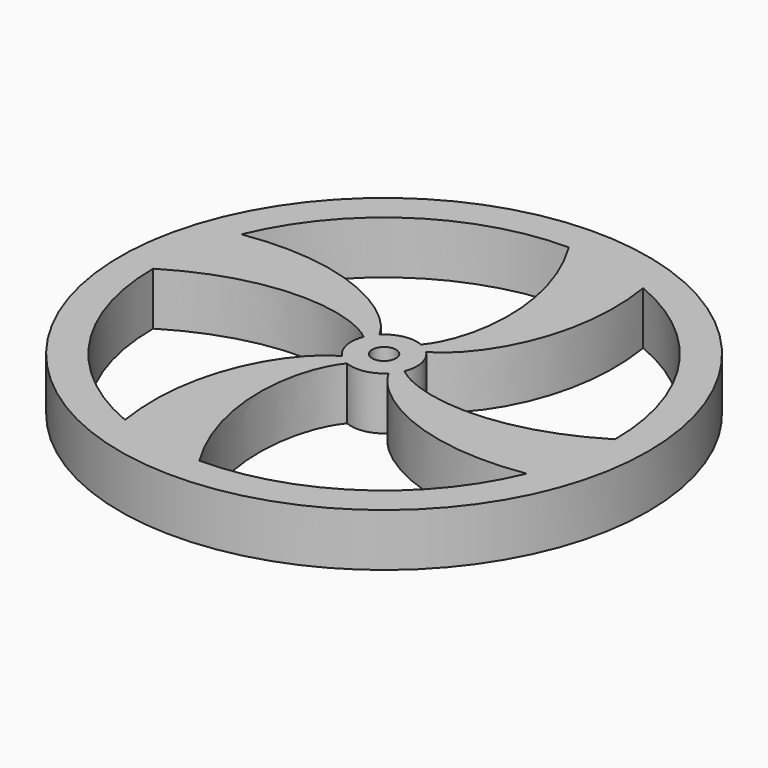
from build123d import *

# Parameters (mm, degrees)
F0_R     = 20
F0_R_2   = 0.9
F1_DEPTH = 4


with BuildPart() as f1:
    # F0 (on Top) → F1 (new body)
    with BuildSketch(Plane.XY):
        Circle(F0_R)
        with BuildLine():
            ThreePointArc((-16.1673680712, 6.6982243655), (-9.7219101416, 14.5510983502), (0, 17.5))
            add(Edge.make_bspline(
                [(0, 17.5), (4.0351947292, 10.8956713768), (2.8402573141, 4.5637440123), (0.9567085809, 2.3096988313)],
                knots=[0, 0, 0, 0, 0.6747802814, 0.6747802814, 0.6747802814, 0.6747802814], degree=3))
            add(Edge.make_bspline(
                [(1.05334234, 1.483872858), (1.0137768965, 1.7486550509), (0.9849575618, 2.0237015142), (0.9567085809, 2.3096988313)],
                knots=[0.9279449305, 0.9279449305, 0.9279449305, 0.9279449305, 1, 1, 1, 1], degree=3))
            add(Edge.make_bspline(
                [(1.7677669525, 1.7677669535), (1.7677118309, 1.7677381162), (1.5223929609, 1.6394048238), (1.2852910821, 1.5468737836), (1.0533423393, 1.4838728598)],
                knots=[0.6747713742, 0.6747713742, 0.6747713742, 0.6747713742, 0.6747856641, 0.7383691109, 0.7383691109, 0.7383691109, 0.7383691109], degree=3))
            add(Edge.make_bspline(
                [(1.76803561, 1.7679075162), (1.7679460564, 1.7678606572), (1.7678565039, 1.7678138029), (1.7677669525, 1.7677669535)],
                knots=[0.6747481586, 0.6747481586, 0.6747481586, 0.6747481586, 0.6747713742, 0.6747713742, 0.6747713742, 0.6747713742], degree=3))
            add(Edge.make_bspline(
                [(6.6984395879, 16.1672789018), (7.8983091219, 8.521720501), (4.3708601286, 3.1298383292), (1.76803561, 1.7679075162)],
                knots=[0, 0, 0, 0, 0.6747481586, 0.6747481586, 0.6747481586, 0.6747481586], degree=3))
            ThreePointArc((6.6984395879, 16.1672789018), (14.5511630598, 9.721813288), (17.5, 0))
            add(Edge.make_bspline(
                [(17.5, 0), (10.8956713768, -4.0351947292), (4.5637440123, -2.8402573141), (2.3096988313, -0.9567085809)],
                knots=[0, 0, 0, 0, 0.6747802814, 0.6747802814, 0.6747802814, 0.6747802814], degree=3))
            add(Edge.make_bspline(
                [(1.4839305002, -1.0533337269), (1.7486949687, -1.0137727139), (2.0237222677, -0.9849555119), (2.3096988313, -0.9567085809)],
                knots=[0.9279501592, 0.9279501592, 0.9279501592, 0.9279501592, 1, 1, 1, 1], degree=3))
            add(Edge.make_bspline(
                [(1.767766953, -1.767766953), (1.7677424454, -1.767720101), (1.639424724, -1.5224005371), (1.5469125425, -1.2852951635), (1.483930502, -1.0533337262)],
                knots=[0.6747683451, 0.6747683451, 0.6747683451, 0.6747683451, 0.674780491, 0.7383651842, 0.7383651842, 0.7383651842, 0.7383651842], degree=3))
            add(Edge.make_bspline(
                [(1.7679075011, -1.7680356179), (1.767860647, -1.7679460618), (1.7678137976, -1.7678565068), (1.767766953, -1.767766953)],
                knots=[0.6747451292, 0.6747451292, 0.6747451292, 0.6747451292, 0.6747683451, 0.6747683451, 0.6747683451, 0.6747683451], degree=3))
            add(Edge.make_bspline(
                [(16.1673680713, -6.6982243654), (8.5218439975, -7.8980885198), (3.1296734519, -4.3708895859), (1.7679075011, -1.7680356179)],
                knots=[0, 0, 0, 0, 0.6747451292, 0.6747451292, 0.6747451292, 0.6747451292], degree=3))
            ThreePointArc((16.1673680713, -6.6982243654), (9.7219101417, -14.5510983502), (0, -17.5))
            add(Edge.make_bspline(
                [(0, -17.5), (-4.0351947292, -10.8956713768), (-2.8402573141, -4.5637440123), (-0.9567085809, -2.3096988313)],
                knots=[0, 0, 0, 0, 0.6747802814, 0.6747802814, 0.6747802814, 0.6747802814], degree=3))
            add(Edge.make_bspline(
                [(-1.0533337269, -1.4839305003), (-1.0137727139, -1.7486949687), (-0.9849555119, -2.0237222677), (-0.9567085809, -2.3096988313)],
                knots=[0.9279501592, 0.9279501592, 0.9279501592, 0.9279501592, 1, 1, 1, 1], degree=3))
            add(Edge.make_bspline(
                [(-1.767766953, -1.767766953), (-1.7677201011, -1.7677424454), (-1.5224005372, -1.639424724), (-1.2852951635, -1.5469125425), (-1.0533337262, -1.483930502)],
                knots=[0.6747683451, 0.6747683451, 0.6747683451, 0.6747683451, 0.674780491, 0.7383651842, 0.7383651842, 0.7383651842, 0.7383651842], degree=3))
            add(Edge.make_bspline(
                [(-1.7680356179, -1.7679075011), (-1.7679460618, -1.767860647), (-1.7678565068, -1.7678137976), (-1.767766953, -1.767766953)],
                knots=[0.6747451293, 0.6747451293, 0.6747451293, 0.6747451293, 0.6747683451, 0.6747683451, 0.6747683451, 0.6747683451], degree=3))
            add(Edge.make_bspline(
                [(-6.6982243654, -16.1673680712), (-7.8980885199, -8.5218439973), (-4.3708895859, -3.1296734518), (-1.7680356179, -1.7679075011)],
                knots=[0, 0, 0, 0, 0.6747451293, 0.6747451293, 0.6747451293, 0.6747451293], degree=3))
            ThreePointArc((-6.6982243654, -16.1673680712), (-14.5510983502, -9.7219101417), (-17.5, 0))
            add(Edge.make_bspline(
                [(-17.5, 0), (-10.8956713768, 4.0351947292), (-4.5637440123, 2.8402573141), (-2.3096988313, 0.9567085809)],
                knots=[0, 0, 0, 0, 0.6747802814, 0.6747802814, 0.6747802814, 0.6747802814], degree=3))
            add(Edge.make_bspline(
                [(-1.4839305003, 1.0533337269), (-1.7486949687, 1.0137727139), (-2.0237222677, 0.9849555119), (-2.3096988313, 0.9567085809)],
                knots=[0.9279501592, 0.9279501592, 0.9279501592, 0.9279501592, 1, 1, 1, 1], degree=3))
            add(Edge.make_bspline(
                [(-1.767766953, 1.767766953), (-1.7677424454, 1.7677201011), (-1.6394247241, 1.5224005372), (-1.5469125425, 1.2852951636), (-1.4839305021, 1.0533337262)],
                knots=[0.6747683451, 0.6747683451, 0.6747683451, 0.6747683451, 0.674780491, 0.7383651842, 0.7383651842, 0.7383651842, 0.7383651842], degree=3))
            add(Edge.make_bspline(
                [(-16.1673680712, 6.6982243655), (-8.5215809386, 7.8981298036), (-3.1293023988, 4.3706468604), (-1.767766953, 1.767766953)],
                knots=[0, 0, 0, 0, 0.6747683451, 0.6747683451, 0.6747683451, 0.6747683451], degree=3))
        make_face(mode=Mode.SUBTRACT)
        with BuildLine():
            add(Edge.make_bspline(
                [(1.05334234, 1.483872858), (1.0137768965, 1.7486550509), (0.9849575618, 2.0237015142), (0.9567085809, 2.3096988313)],
                knots=[0.9279449305, 0.9279449305, 0.9279449305, 0.9279449305, 1, 1, 1, 1], degree=3))
            add(Edge.make_bspline(
                [(0.9567085809, 2.3096988313), (0.5925556194, 1.873916516), (0.202663868, 1.5905565475), (-0.2170414882, 1.3992266891)],
                knots=[0.6747802814, 0.6747802814, 0.6747802814, 0.6747802814, 0.8052378764, 0.8052378764, 0.8052378764, 0.8052378764], degree=3))
            add(Edge.make_bspline(
                [(1.0533423393, 1.4838728598), (0.6188058723, 1.3658459262), (0.2021683226, 1.3513874939), (-0.2170414882, 1.3992266891)],
                knots=[0.7383691109, 0.7383691109, 0.7383691109, 0.7383691109, 0.8574873522, 0.8574873522, 0.8574873522, 0.8574873522], degree=3))
        make_face()
        with BuildLine():
            add(Edge.make_bspline(
                [(0.9567085809, 2.3096988313), (0.5925556194, 1.873916516), (0.202663868, 1.5905565475), (-0.2170414882, 1.3992266891)],
                knots=[0.6747802814, 0.6747802814, 0.6747802814, 0.6747802814, 0.8052378764, 0.8052378764, 0.8052378764, 0.8052378764], degree=3))
            ThreePointArc((0.9567085809, 2.3096988313), (-0.4877258051, 2.451963201), (-1.767766953, 1.767766953))
            add(Edge.make_bspline(
                [(-0.2170414882, 1.3992266891), (-0.7185826414, 1.4564613351), (-1.2238056379, 1.6028665997), (-1.767766953, 1.767766953)],
                knots=[0.8574873522, 0.8574873522, 0.8574873522, 0.8574873522, 1, 1, 1, 1], degree=3))
        make_face()
        with BuildLine():
            add(Edge.make_bspline(
                [(-0.2170414882, 1.3992266891), (-0.7185826414, 1.4564613351), (-1.2238056379, 1.6028665997), (-1.767766953, 1.767766953)],
                knots=[0.8574873522, 0.8574873522, 0.8574873522, 0.8574873522, 1, 1, 1, 1], degree=3))
            add(Edge.make_bspline(
                [(-1.767766953, 1.767766953), (-1.7677424454, 1.7677201011), (-1.6394247241, 1.5224005372), (-1.5469125425, 1.2852951636), (-1.4839305021, 1.0533337262)],
                knots=[0.6747683451, 0.6747683451, 0.6747683451, 0.6747683451, 0.674780491, 0.7383651842, 0.7383651842, 0.7383651842, 0.7383651842], degree=3))
            add(Edge.make_bspline(
                [(-0.2170414882, 1.3992266891), (-0.6118287934, 1.21925615), (-1.0329947036, 1.1207123938), (-1.4839305003, 1.0533337269)],
                knots=[0.8052378764, 0.8052378764, 0.8052378764, 0.8052378764, 0.9279501592, 0.9279501592, 0.9279501592, 0.9279501592], degree=3))
        make_face()
        with BuildLine():
            add(Edge.make_bspline(
                [(1.0533423393, 1.4838728598), (0.6188058723, 1.3658459262), (0.2021683226, 1.3513874939), (-0.2170414882, 1.3992266891)],
                knots=[0.7383691109, 0.7383691109, 0.7383691109, 0.7383691109, 0.8574873522, 0.8574873522, 0.8574873522, 0.8574873522], degree=3))
            add(Edge.make_bspline(
                [(-0.2170414882, 1.3992266891), (-0.6118287934, 1.21925615), (-1.0329947036, 1.1207123938), (-1.4839305003, 1.0533337269)],
                knots=[0.8052378764, 0.8052378764, 0.8052378764, 0.8052378764, 0.9279501592, 0.9279501592, 0.9279501592, 0.9279501592], degree=3))
            add(Edge.make_bspline(
                [(-1.4839305021, 1.0533337262), (-1.3659750292, 0.6189063747), (-1.3515357612, 0.2023627588), (-1.3993629137, -0.2167427021)],
                knots=[0.7383651842, 0.7383651842, 0.7383651842, 0.7383651842, 0.8574493311, 0.8574493311, 0.8574493311, 0.8574493311], degree=3))
            add(Edge.make_bspline(
                [(-1.3993629137, -0.2167427021), (-1.2193058732, -0.6116162916), (-1.1207293921, -1.0328809414), (-1.0533337269, -1.4839305003)],
                knots=[0.8052069185, 0.8052069185, 0.8052069185, 0.8052069185, 0.9279501592, 0.9279501592, 0.9279501592, 0.9279501592], degree=3))
            add(Edge.make_bspline(
                [(-1.0533337262, -1.483930502), (-0.6189063746, -1.3659750292), (-0.2023627587, -1.3515357612), (0.2167427022, -1.3993629136)],
                knots=[0.7383651842, 0.7383651842, 0.7383651842, 0.7383651842, 0.8574493311, 0.8574493311, 0.8574493311, 0.8574493311], degree=3))
            add(Edge.make_bspline(
                [(0.2167427022, -1.3993629136), (0.6116162917, -1.2193058732), (1.0328809414, -1.1207293921), (1.4839305002, -1.0533337269)],
                knots=[0.8052069185, 0.8052069185, 0.8052069185, 0.8052069185, 0.9279501592, 0.9279501592, 0.9279501592, 0.9279501592], degree=3))
            add(Edge.make_bspline(
                [(1.483930502, -1.0533337262), (1.3659750291, -0.6189063746), (1.3515357611, -0.2023627586), (1.3993629136, 0.2167427023)],
                knots=[0.7383651842, 0.7383651842, 0.7383651842, 0.7383651842, 0.8574493311, 0.8574493311, 0.8574493311, 0.8574493311], degree=3))
            add(Edge.make_bspline(
                [(1.3993629136, 0.2167427023), (1.2193135434, 0.6115994707), (1.1207377907, 1.0328450508), (1.05334234, 1.483872858)],
                knots=[0.8052069185, 0.8052069185, 0.8052069185, 0.8052069185, 0.9279449305, 0.9279449305, 0.9279449305, 0.9279449305], degree=3))
        make_face()
        Circle(F0_R_2, mode=Mode.SUBTRACT)
        with BuildLine():
            add(Edge.make_bspline(
                [(1.7677669525, 1.7677669535), (1.7677118309, 1.7677381162), (1.5223929609, 1.6394048238), (1.2852910821, 1.5468737836), (1.0533423393, 1.4838728598)],
                knots=[0.6747713742, 0.6747713742, 0.6747713742, 0.6747713742, 0.6747856641, 0.7383691109, 0.7383691109, 0.7383691109, 0.7383691109], degree=3))
            add(Edge.make_bspline(
                [(1.3993629136, 0.2167427023), (1.2193135434, 0.6115994707), (1.1207377907, 1.0328450508), (1.05334234, 1.483872858)],
                knots=[0.8052069185, 0.8052069185, 0.8052069185, 0.8052069185, 0.9279449305, 0.9279449305, 0.9279449305, 0.9279449305], degree=3))
            add(Edge.make_bspline(
                [(1.3993629136, 0.2167427023), (1.45660379, 0.7183398629), (1.6030349201, 1.2236066033), (1.7679404268, 1.7675934622)],
                knots=[0.8574493311, 0.8574493311, 0.8574493311, 0.8574493311, 0.9999725754, 0.9999725754, 0.9999725754, 0.9999725754], degree=3))
            ThreePointArc((1.7679404268, 1.7675934622), (1.7678536918, 1.7676802099), (1.7677669525, 1.7677669535))
        make_face()
        with BuildLine():
            add(Edge.make_bspline(
                [(-1.4839305021, 1.0533337262), (-1.3659750292, 0.6189063747), (-1.3515357612, 0.2023627588), (-1.3993629137, -0.2167427021)],
                knots=[0.7383651842, 0.7383651842, 0.7383651842, 0.7383651842, 0.8574493311, 0.8574493311, 0.8574493311, 0.8574493311], degree=3))
            add(Edge.make_bspline(
                [(-1.4839305003, 1.0533337269), (-1.7486949687, 1.0137727139), (-2.0237222677, 0.9849555119), (-2.3096988313, 0.9567085809)],
                knots=[0.9279501592, 0.9279501592, 0.9279501592, 0.9279501592, 1, 1, 1, 1], degree=3))
            add(Edge.make_bspline(
                [(-2.3096988313, 0.9567085809), (-1.8740199281, 0.5926420338), (-1.59069104, 0.2028489109), (-1.3993629137, -0.2167427021)],
                knots=[0.6747802814, 0.6747802814, 0.6747802814, 0.6747802814, 0.8052069185, 0.8052069185, 0.8052069185, 0.8052069185], degree=3))
        make_face()
        with BuildLine():
            add(Edge.make_bspline(
                [(1.3993629136, 0.2167427023), (1.45660379, 0.7183398629), (1.6030349201, 1.2236066033), (1.7679404268, 1.7675934622)],
                knots=[0.8574493311, 0.8574493311, 0.8574493311, 0.8574493311, 0.9999725754, 0.9999725754, 0.9999725754, 0.9999725754], degree=3))
            add(Edge.make_bspline(
                [(2.3096988313, -0.9567085809), (1.874019928, -0.5926420337), (1.5906910399, -0.2028489108), (1.3993629136, 0.2167427023)],
                knots=[0.6747802814, 0.6747802814, 0.6747802814, 0.6747802814, 0.8052069185, 0.8052069185, 0.8052069185, 0.8052069185], degree=3))
            ThreePointArc((2.3096988313, -0.9567085809), (2.4519871299, 0.487605491), (1.7679404268, 1.7675934622))
        make_face()
        with BuildLine():
            add(Edge.make_bspline(
                [(2.3096988313, -0.9567085809), (1.874019928, -0.5926420337), (1.5906910399, -0.2028489108), (1.3993629136, 0.2167427023)],
                knots=[0.6747802814, 0.6747802814, 0.6747802814, 0.6747802814, 0.8052069185, 0.8052069185, 0.8052069185, 0.8052069185], degree=3))
            add(Edge.make_bspline(
                [(1.483930502, -1.0533337262), (1.3659750291, -0.6189063746), (1.3515357611, -0.2023627586), (1.3993629136, 0.2167427023)],
                knots=[0.7383651842, 0.7383651842, 0.7383651842, 0.7383651842, 0.8574493311, 0.8574493311, 0.8574493311, 0.8574493311], degree=3))
            add(Edge.make_bspline(
                [(1.4839305002, -1.0533337269), (1.7486949687, -1.0137727139), (2.0237222677, -0.9849555119), (2.3096988313, -0.9567085809)],
                knots=[0.9279501592, 0.9279501592, 0.9279501592, 0.9279501592, 1, 1, 1, 1], degree=3))
        make_face()
        with BuildLine():
            add(Edge.make_bspline(
                [(-2.3096988313, 0.9567085809), (-1.8740199281, 0.5926420338), (-1.59069104, 0.2028489109), (-1.3993629137, -0.2167427021)],
                knots=[0.6747802814, 0.6747802814, 0.6747802814, 0.6747802814, 0.8052069185, 0.8052069185, 0.8052069185, 0.8052069185], degree=3))
            ThreePointArc((-2.3096988313, 0.9567085809), (-2.4519871299, -0.4876054909), (-1.7679404269, -1.767593462))
            add(Edge.make_bspline(
                [(-1.3993629137, -0.2167427021), (-1.4566037901, -0.7183398627), (-1.6030349202, -1.2236066032), (-1.7679404269, -1.767593462)],
                knots=[0.8574493311, 0.8574493311, 0.8574493311, 0.8574493311, 0.9999725754, 0.9999725754, 0.9999725754, 0.9999725754], degree=3))
        make_face()
        with BuildLine():
            add(Edge.make_bspline(
                [(-1.3993629137, -0.2167427021), (-1.2193058732, -0.6116162916), (-1.1207293921, -1.0328809414), (-1.0533337269, -1.4839305003)],
                knots=[0.8052069185, 0.8052069185, 0.8052069185, 0.8052069185, 0.9279501592, 0.9279501592, 0.9279501592, 0.9279501592], degree=3))
            add(Edge.make_bspline(
                [(-1.3993629137, -0.2167427021), (-1.4566037901, -0.7183398627), (-1.6030349202, -1.2236066032), (-1.7679404269, -1.767593462)],
                knots=[0.8574493311, 0.8574493311, 0.8574493311, 0.8574493311, 0.9999725754, 0.9999725754, 0.9999725754, 0.9999725754], degree=3))
            ThreePointArc((-1.7679404269, -1.767593462), (-1.7678536921, -1.7676802097), (-1.767766953, -1.767766953))
            add(Edge.make_bspline(
                [(-1.767766953, -1.767766953), (-1.7677201011, -1.7677424454), (-1.5224005372, -1.639424724), (-1.2852951635, -1.5469125425), (-1.0533337262, -1.483930502)],
                knots=[0.6747683451, 0.6747683451, 0.6747683451, 0.6747683451, 0.674780491, 0.7383651842, 0.7383651842, 0.7383651842, 0.7383651842], degree=3))
        make_face()
        with BuildLine():
            add(Edge.make_bspline(
                [(1.767766953, -1.767766953), (1.7677424454, -1.767720101), (1.639424724, -1.5224005371), (1.5469125425, -1.2852951635), (1.483930502, -1.0533337262)],
                knots=[0.6747683451, 0.6747683451, 0.6747683451, 0.6747683451, 0.674780491, 0.7383651842, 0.7383651842, 0.7383651842, 0.7383651842], degree=3))
            add(Edge.make_bspline(
                [(0.2167427022, -1.3993629136), (0.6116162917, -1.2193058732), (1.0328809414, -1.1207293921), (1.4839305002, -1.0533337269)],
                knots=[0.8052069185, 0.8052069185, 0.8052069185, 0.8052069185, 0.9279501592, 0.9279501592, 0.9279501592, 0.9279501592], degree=3))
            add(Edge.make_bspline(
                [(0.2167427022, -1.3993629136), (0.7183398628, -1.45660379), (1.2236066033, -1.6030349201), (1.7675934621, -1.7679404269)],
                knots=[0.8574493311, 0.8574493311, 0.8574493311, 0.8574493311, 0.9999725754, 0.9999725754, 0.9999725754, 0.9999725754], degree=3))
            ThreePointArc((1.7675934621, -1.7679404269), (1.7676802097, -1.767853692), (1.767766953, -1.767766953))
        make_face()
        with BuildLine():
            add(Edge.make_bspline(
                [(-1.0533337262, -1.483930502), (-0.6189063746, -1.3659750292), (-0.2023627587, -1.3515357612), (0.2167427022, -1.3993629136)],
                knots=[0.7383651842, 0.7383651842, 0.7383651842, 0.7383651842, 0.8574493311, 0.8574493311, 0.8574493311, 0.8574493311], degree=3))
            add(Edge.make_bspline(
                [(-1.0533337269, -1.4839305003), (-1.0137727139, -1.7486949687), (-0.9849555119, -2.0237222677), (-0.9567085809, -2.3096988313)],
                knots=[0.9279501592, 0.9279501592, 0.9279501592, 0.9279501592, 1, 1, 1, 1], degree=3))
            add(Edge.make_bspline(
                [(-0.9567085809, -2.3096988313), (-0.5926420337, -1.8740199281), (-0.2028489108, -1.59069104), (0.2167427022, -1.3993629136)],
                knots=[0.6747802814, 0.6747802814, 0.6747802814, 0.6747802814, 0.8052069185, 0.8052069185, 0.8052069185, 0.8052069185], degree=3))
        make_face()
        with BuildLine():
            add(Edge.make_bspline(
                [(0.2167427022, -1.3993629136), (0.7183398628, -1.45660379), (1.2236066033, -1.6030349201), (1.7675934621, -1.7679404269)],
                knots=[0.8574493311, 0.8574493311, 0.8574493311, 0.8574493311, 0.9999725754, 0.9999725754, 0.9999725754, 0.9999725754], degree=3))
            add(Edge.make_bspline(
                [(-0.9567085809, -2.3096988313), (-0.5926420337, -1.8740199281), (-0.2028489108, -1.59069104), (0.2167427022, -1.3993629136)],
                knots=[0.6747802814, 0.6747802814, 0.6747802814, 0.6747802814, 0.8052069185, 0.8052069185, 0.8052069185, 0.8052069185], degree=3))
            ThreePointArc((-0.9567085809, -2.3096988313), (0.487605491, -2.4519871299), (1.7675934621, -1.7679404269))
        make_face()
    extrude(amount=F1_DEPTH)


solid = f1.part
